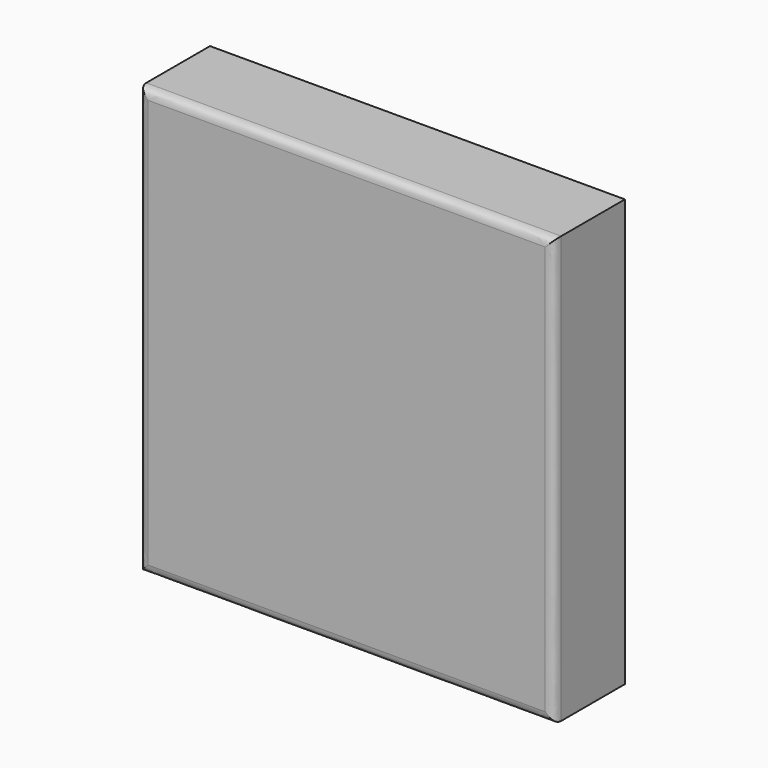
from build123d import *

# Parameters (mm, degrees)
F0_W        = 119.0486699343
F0_H        = 122.4547103047
F1_DEPTH    = 25.4
F2_T1_DEPTH = 131.7486699343
F2_T3_DEPTH = 135.1547103047
F3_T        = -5.08


# Not quite as in the source:
# - a fillet or chamfer that OpenCascade refuses, or shapes differently, is made with other operations: its cross-section is extruded or revolved along the edge and cut away or added


with BuildPart() as f1:
    # F0 (on Front) → F1 (new body)
    with BuildSketch(Plane.XZ):
        Rectangle(F0_W, F0_H)
    extrude(amount=F1_DEPTH)

    # F2: fillet of radius 2.54 on 4 edges, made by hand

    # F2_s2 → F2_t1 (cut)
    with BuildSketch(Plane.YZ.offset(-65.8743349671)):
        with BuildLine():
            add(Edge.make_bspline(
                [(-22.86, 61.2273551524), (-25.4, 61.2273551524), (-25.4, 58.6873551524)],
                knots=[0, 0, 0, 1, 1, 1], degree=2, weights=[1, 1, 1]))
            Line((-25.4, 58.6873551524), (-25.4, 61.2273551524))
            Line((-25.4, 61.2273551524), (-22.86, 61.2273551524))
        make_face()
        with BuildLine():
            add(Edge.make_bspline(
                [(-22.86, -61.2273551524), (-25.4, -61.2273551524), (-25.4, -58.6873551524)],
                knots=[0, 0, 0, 1, 1, 1], degree=2, weights=[1, 1, 1]))
            Line((-25.4, -58.6873551524), (-25.4, -61.2273551524))
            Line((-25.4, -61.2273551524), (-22.86, -61.2273551524))
        make_face()
    extrude(amount=F2_T1_DEPTH, mode=Mode.SUBTRACT)

    # F2_s4 → F2_t3 (cut)
    with BuildSketch(Plane.XY.offset(-67.5773551524)):
        with BuildLine():
            add(Edge.make_bspline(
                [(-59.5243349671, -22.86), (-59.5243349671, -25.4), (-56.9843349671, -25.4)],
                knots=[0, 0, 0, 1, 1, 1], degree=2, weights=[1, 1, 1]))
            Line((-56.9843349671, -25.4), (-59.5243349671, -25.4))
            Line((-59.5243349671, -25.4), (-59.5243349671, -22.86))
        make_face()
        with BuildLine():
            add(Edge.make_bspline(
                [(59.5243349671, -22.86), (59.5243349671, -25.4), (56.9843349671, -25.4)],
                knots=[0, 0, 0, 1, 1, 1], degree=2, weights=[1, 1, 1]))
            Line((56.9843349671, -25.4), (59.5243349671, -25.4))
            Line((59.5243349671, -25.4), (59.5243349671, -22.86))
        make_face()
    extrude(amount=F2_T3_DEPTH, mode=Mode.SUBTRACT)

    # F3
    f3_openings = [f1.faces().sort_by_distance(p)[0] for p in [
        (0, 0, 0),
    ]]
    offset(amount=F3_T, openings=f3_openings)


solid = f1.part
